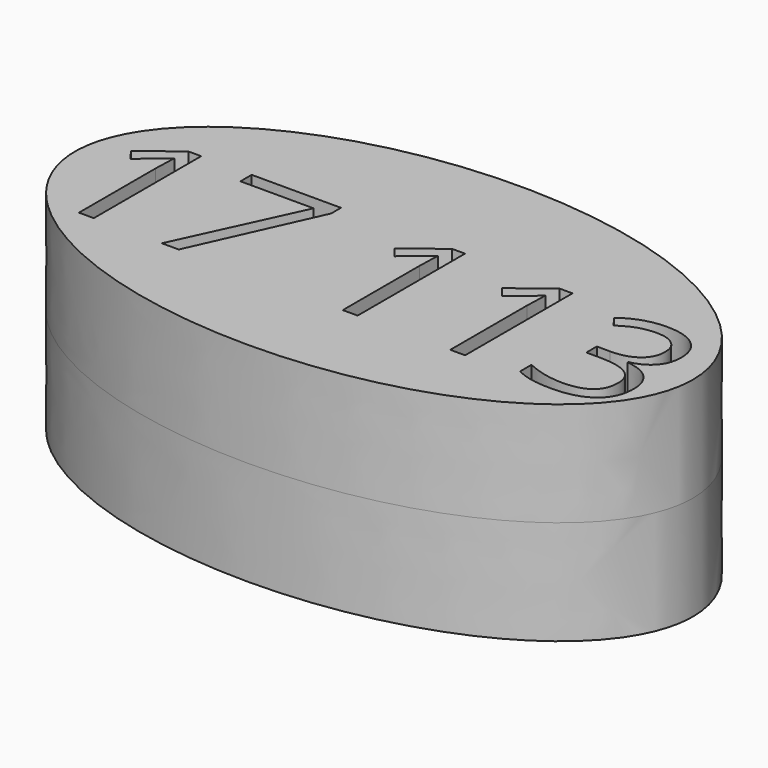
from build123d import *

# Parameters (mm, degrees)
F1_DEPTH     = 25.4
F2_DEPTH     = 25.4
F3_DEPTH     = 25.4
F4_TEXT_SIZE = 45.7901016085
F5_DEPTH     = 25.4


# Not quite as in the source:
# - Text() gives the source's letters only with a copy of the font that has no kerning and outlines rounded to 1/6400 em; it was checked with that copy


with BuildPart() as f1:
    # F0 (on Top) → F1 (new body)
    with BuildSketch(Plane.XY):
        with BuildLine():
            add(Edge.make_bspline(
                [(75.2484053373, 0), (75.2484053373, 72.2025148046), (-37.6242026687, 36.1012574023), (-150.4968106747, 0), (-37.6242026687, -36.1012574023), (75.2484053373, -72.2025148046), (75.2484053373, 0)],
                knots=[0, 0, 0, 2.0943951024, 2.0943951024, 4.1887902048, 4.1887902048, 6.2831853072, 6.2831853072, 6.2831853072], degree=2, weights=[1, 0.5, 1, 0.5, 1, 0.5, 1]))
        make_face()
    extrude(amount=F1_DEPTH)

    # F2 (add): a face of the model
    f2_faces = [f1.faces().sort_by_distance(p)[0] for p in [
        (0.3996219625, 0, 25.4),
    ]]
    extrude(f2_faces, amount=-F2_DEPTH)

    # F3 (add): a face of the model
    f3_faces = [f1.faces().sort_by_distance(p)[0] for p in [
        (0.3996219625, 0, 25.4),
    ]]
    extrude(f3_faces, amount=F3_DEPTH)

    # F4 (on face) → F5 (cut)
    with BuildSketch(Plane.XY.offset(50.8)):
        with Locations((-71.2799287867, -19.2318474874)):
            Text('17 113', F4_TEXT_SIZE, font='Open Sans', text_align=(TextAlign.LEFT, TextAlign.BOTTOM))
    extrude(amount=-F5_DEPTH, mode=Mode.SUBTRACT)


solid = f1.part
